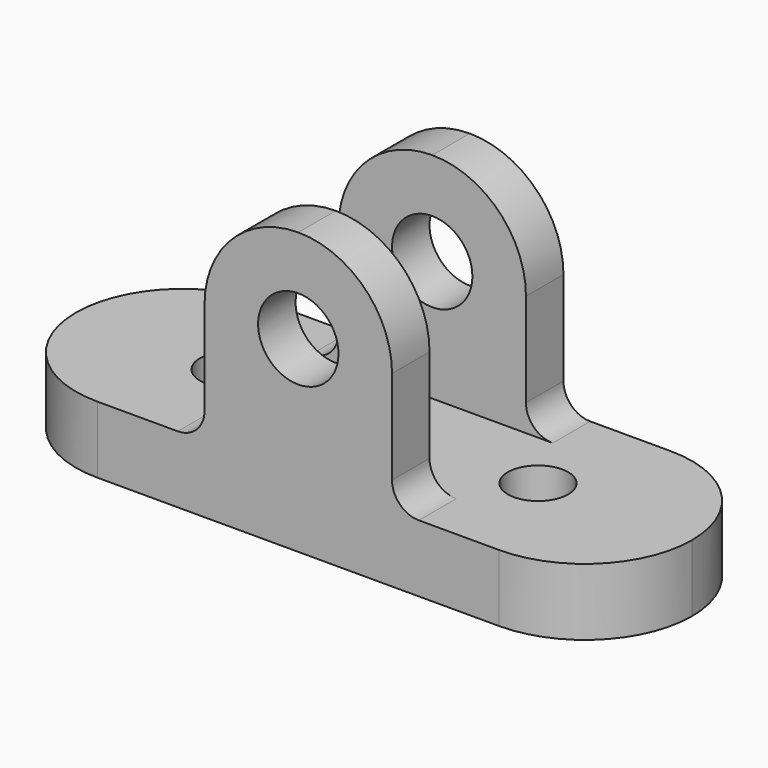
from build123d import *

# Parameters (mm, degrees)
F0_W     = 14
F0_H     = 7
F1_DEPTH = 10
F2_R     = 15.99999
F3_D     = 9
F4_DEPTH = 42
F5_R     = 4
F7_D     = 12
F8_R     = 13.99999


# Not quite as in the source:
# - a fillet or chamfer is up to 0.001 mm smaller than in the source, because OpenCascade refuses the exact size


with BuildPart() as f1:
    # F0 (on Top) → F1 (new body)
    with BuildSketch(Plane.XY):
        Polygon((46, 0), (46, 16), (14, 16), (14, 9), (0, 9), (0, 0), (23, 0), align=None)
        with Locations((7, 12.5)):
            Rectangle(F0_W, F0_H)
        Polygon((46, -16), (46, 0), (23, 0), (0, 0), (0, -9), (14, -9), (14, -16), align=None)
        with Locations((-7, 12.5)):
            Rectangle(F0_W, F0_H)
        Polygon((-14, 9), (-14, 16), (-46, 16), (-46, 0), (-23, 0), (0, 0), (0, 9), align=None)
        with Locations((7, -12.5)):
            Rectangle(F0_W, F0_H)
        Polygon((0, -9), (0, 0), (-23, 0), (-46, 0), (-46, -16), (-14, -16), (-14, -9), align=None)
        with Locations((-7, -12.5)):
            Rectangle(F0_W, F0_H)
    extrude(amount=F1_DEPTH)

    # F2 (radius 16 in the source; OpenCascade refuses exactly that, so slightly less here)
    f2_edges = [f1.edges().sort_by_distance(p)[0] for p in [
        (-46, -16, 5),
        (-46, 16, 5),
        (46, 16, 5),
        (46, -16, 5),
    ]]
    fillet(f2_edges, radius=F2_R)

    # F3 (through all)
    with Locations(Plane(origin=(0, 0, 0), x_dir=(1, 0, 0), z_dir=(0, 0, -1))):
        with Locations((23, 0), (-23, 0)):
            Hole(F3_D / 2)

    # F0 (on Top) → F4 (join)
    with BuildSketch(Plane.XY):
        with Locations((-7, -12.5)):
            Rectangle(F0_W, F0_H)
        with Locations((7, -12.5)):
            Rectangle(F0_W, F0_H)
        with Locations((-7, 12.5)):
            Rectangle(F0_W, F0_H)
        with Locations((7, 12.5)):
            Rectangle(F0_W, F0_H)
    extrude(amount=F4_DEPTH)

    # F5
    f5_edges = [f1.edges().sort_by_distance(p)[0] for p in [
        (14, 12.5, 10),
        (14, -12.5, 10),
        (-14, 12.5, 10),
        (-14, -12.5, 10),
    ]]
    fillet(f5_edges, radius=F5_R)

    # F7 (through all)
    with Locations(Plane(origin=(0, 16, 0), x_dir=(-1, 0, 0), z_dir=(0, 1, 0))):
        with Locations((0, 28)):
            Hole(F7_D / 2)

    # F8 (radius 14 in the source; OpenCascade refuses exactly that, so slightly less here)
    f8_edges = [f1.edges().sort_by_distance(p)[0] for p in [
        (14, 12.5, 42),
        (-14, 12.5, 42),
        (14, -12.5, 42),
        (-14, -12.5, 42),
    ]]
    fillet(f8_edges, radius=F8_R)


solid = f1.part
